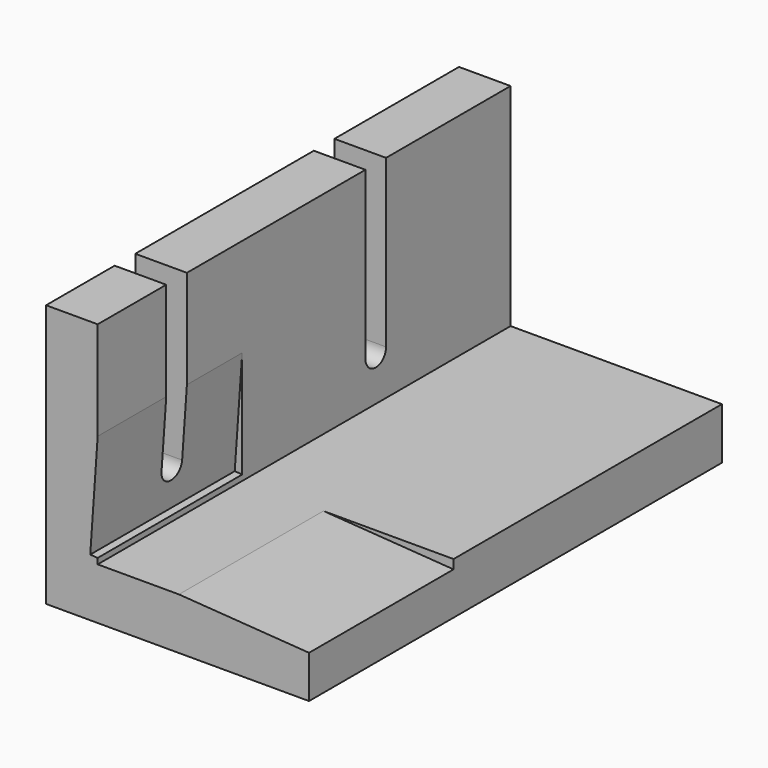
from build123d import *

# Parameters (mm, degrees)
F0_W     = 64.7085476667
F0_H     = 64.7085476667
F1_DEPTH = 127
F2_W     = 52.0085476667
F2_H     = 52.0085476667
F3_DEPTH = 127.001
F5_DEPTH = 44.45
F6_W     = 6.35
F6_H     = 24.2487721393
F7_DEPTH = 12.701
F9_DEPTH = 12.7


# Not quite as in the source:
# - a feature names something its author has since deleted; it is built from what else it names


with BuildPart() as f1:
    # F0 (on Front) → F1 (new body)
    with BuildSketch(Plane.XZ):
        with Locations((-1.2904843315, -7.374192588)):
            Rectangle(F0_W, F0_H)
    extrude(amount=-F1_DEPTH)

    # F2 (on face) → F3 (cut, through all)
    with BuildSketch(Plane(origin=(0, 127, 0), x_dir=(-1, 0, 0), z_dir=(0, 1, 0))):
        with Locations((-5.0595156685, -1.024192588)):
            Rectangle(F2_W, F2_H)
    extrude(amount=-F3_DEPTH, mode=Mode.SUBTRACT)

    # F4 (on face) → F5 (cut)
    with BuildSketch(Plane.XZ):
        Polygon((31.0637895018, -27.0284664214), (-0.9437288021, -27.0284664214), (31.0637895018, -29.2666501498), align=None)
        Polygon((-20.9447581649, -25.6298581929), (-20.9447581649, 0.731309106), (-22.7791408762, -25.5015856572), align=None)
    extrude(amount=-F5_DEPTH, mode=Mode.SUBTRACT)

    # F6 (on face) → F7 (cut, through all)
    with BuildSketch(Plane.YZ.offset(-20.9447581649)):
        with Locations((24.2636220248, 12.8556951756)):
            Rectangle(F6_W, F6_H)
        with BuildLine():
            Line((27.4386220248, -15.9778556544), (27.4386220248, 0.731309106))
            Line((27.4386220248, 0.731309106), (21.0886220248, 0.731309106))
            Line((21.0886220248, 0.731309106), (21.0886220248, -15.9778556544))
            ThreePointArc((21.0886220248, -15.9778556544), (24.2636220248, -19.1528556544), (27.4386220248, -15.9778556544))
        make_face()
        with BuildLine():
            Line((88.7001905876, 24.9800812453), (82.3501905876, 24.9800812453))
            Line((82.3501905876, 24.9800812453), (82.3501905876, -15.9781904151))
            ThreePointArc((82.3501905876, -15.9781904151), (85.5251905876, -19.1531904151), (88.7001905876, -15.9781904151))
            Line((88.7001905876, -15.9781904151), (88.7001905876, 24.9800812453))
        make_face()
    extrude(amount=-F7_DEPTH, mode=Mode.SUBTRACT)

    # F8 (on face) → F9 (cut)
    with BuildSketch(Plane(origin=(0, 127, 0), x_dir=(-1, 0, 0), z_dir=(0, 1, 0))):
        with BuildLine():
            Line((33.6447581649, -39.7284664214), (33.6447581649, -30.2034664214))
            ThreePointArc((33.6447581649, -30.2034664214), (26.9095660741, -32.9932743306), (24.1197581649, -39.7284664214))
            Line((24.1197581649, -39.7284664214), (33.6447581649, -39.7284664214))
        make_face()
    extrude(amount=-F9_DEPTH, mode=Mode.SUBTRACT)


solid = f1.part
